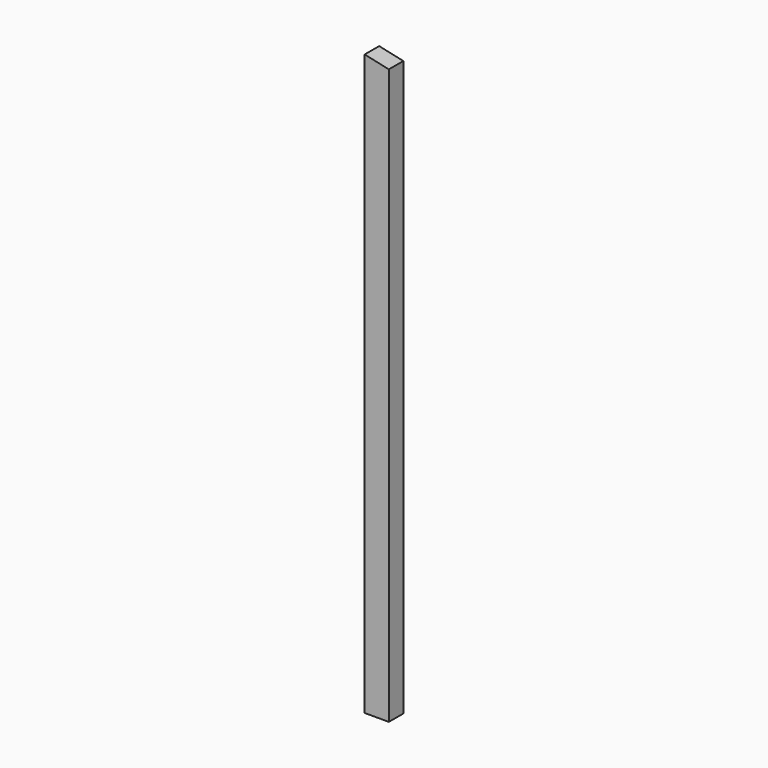
from build123d import *

# Parameters (mm, degrees)
F0_W        = 100
F0_H        = 75
F1_DEPTH    = 2400
F2_T1_DEPTH = 599.7539650252


# Not quite as in the source:
# - a fillet or chamfer that OpenCascade refuses, or shapes differently, is made with other operations: its cross-section is extruded or revolved along the edge and cut away or added


with BuildPart() as f1:
    # F0 (on Top) → F1 (new body)
    with BuildSketch(Plane.XY):
        with Locations((-50, -21.705695812)):
            Rectangle(F0_W, F0_H)
    extrude(amount=-F1_DEPTH)

    # F2: chamfer of 101 x 22.0215613035 on 1 edges, made by hand

    # F2_s2 → F2_t1 (cut)
    with BuildSketch(Plane.XZ.offset(-278.1712867006)):
        Polygon((0, -22.0215613035), (-101, 0), (0, 0), align=None)
    extrude(amount=F2_T1_DEPTH, mode=Mode.SUBTRACT)


solid = f1.part
